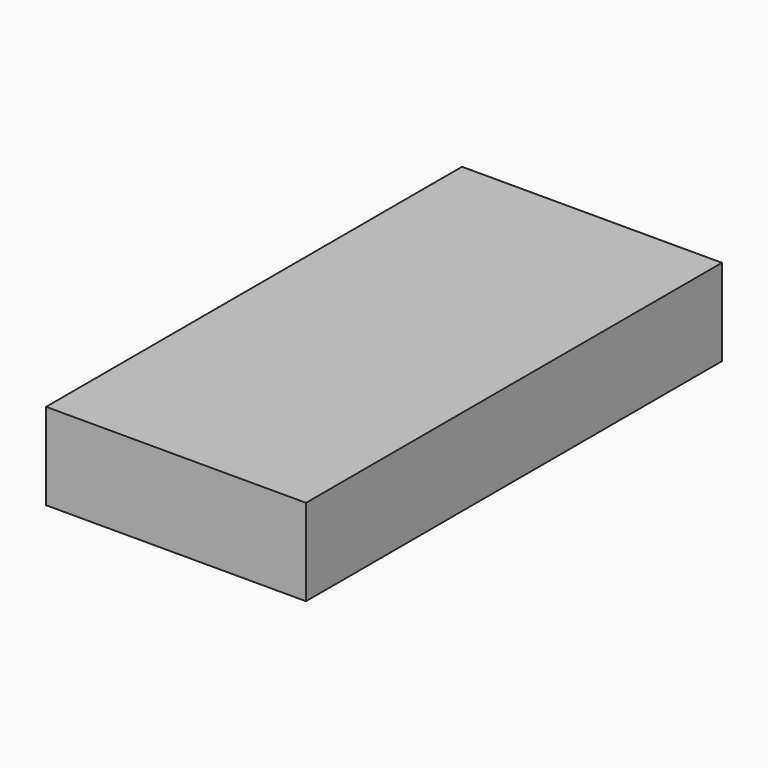
from build123d import *

# Parameters (mm, degrees)
F0_W     = 38.1
F0_H     = 12.7
F2_DEPTH = 38.1


# Not quite as in the source:
# - the program builds the solid bodies; features that only make, move or delete a surface that nothing else refers to are left out


with BuildPart() as f2:
    # F0 (on Front) → F2 (new body, symmetric)
    with BuildSketch(Plane.XZ):
        Rectangle(F0_W, F0_H)
    extrude(amount=F2_DEPTH, both=True)


solid = f2.part
